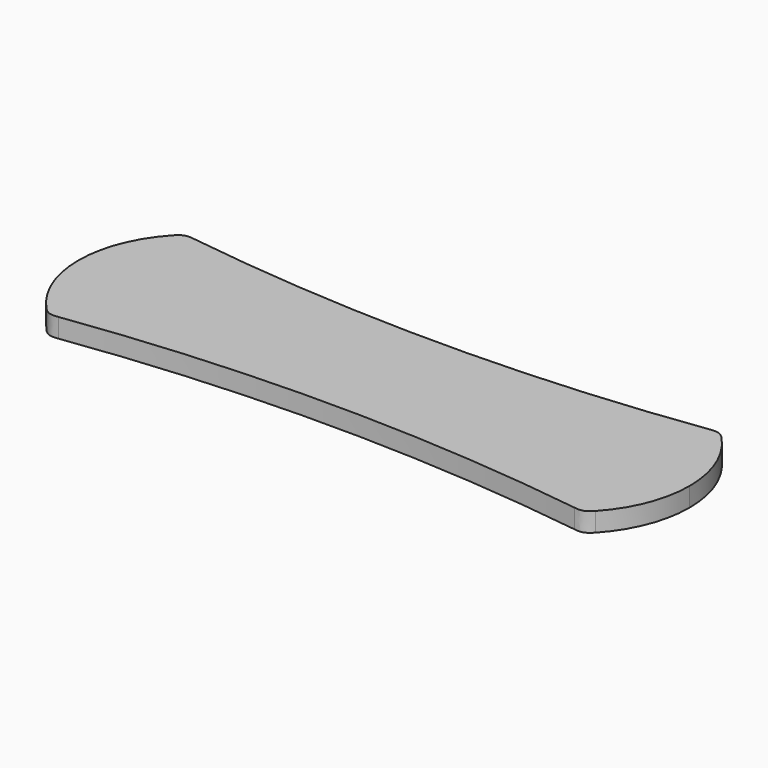
from build123d import *

# Parameters (mm, degrees)
F1_DEPTH    = 25.4
F2_T1_DEPTH = 93.9988541888


# Not quite as in the source:
# - a fillet or chamfer that OpenCascade refuses, or shapes differently, is made with other operations: its cross-section is extruded or revolved along the edge and cut away or added


with BuildPart() as f1:
    # F0 (on Top) → F1 (new body)
    with BuildSketch(Plane.XY):
        with BuildLine():
            ThreePointArc((50.8, 558.8), (13.2719441568, 507.0402470414), (0, 444.5))
            ThreePointArc((0, 444.5), (13.2719441568, 381.9597529586), (50.8, 330.2))
            Line((50.8, 330.2), (50.8, 558.8))
        make_face()
        with BuildLine():
            ThreePointArc((277.2968022896, 536.7332159534), (163.7973759268, 545.1900472484), (50.8, 558.8))
            Line((50.8, 558.8), (50.8, 330.2))
            ThreePointArc((50.8, 330.2), (163.7973759268, 343.8099527516), (277.2968022896, 352.2667840466))
            ThreePointArc((277.2968022896, 352.2667840466), (300.1043048901, 395.8992851393), (307.975, 444.5))
            ThreePointArc((307.975, 444.5), (300.1043048901, 493.1007148607), (277.2968022896, 536.7332159534))
        make_face()
        with BuildLine():
            Line((762, 330.2), (762, 558.8))
            ThreePointArc((762, 558.8), (649.0026240732, 545.1900472484), (535.5031977104, 536.7332159534))
            ThreePointArc((535.5031977104, 536.7332159534), (504.825, 444.5), (535.5031977104, 352.2667840466))
            ThreePointArc((535.5031977104, 352.2667840466), (649.0026240732, 343.8099527516), (762, 330.2))
        make_face()
        with BuildLine():
            ThreePointArc((812.8, 444.5), (799.5280558432, 507.0402470414), (762, 558.8))
            Line((762, 558.8), (762, 330.2))
            ThreePointArc((762, 330.2), (799.5280558432, 381.9597529586), (812.8, 444.5))
        make_face()
        with BuildLine():
            ThreePointArc((535.5031977104, 536.7332159534), (406.4, 533.4), (277.2968022896, 536.7332159534))
            ThreePointArc((277.2968022896, 536.7332159534), (300.1043048901, 493.1007148607), (307.975, 444.5))
            ThreePointArc((307.975, 444.5), (300.1043048901, 395.8992851393), (277.2968022896, 352.2667840466))
            ThreePointArc((277.2968022896, 352.2667840466), (406.4, 355.6), (535.5031977104, 352.2667840466))
            ThreePointArc((535.5031977104, 352.2667840466), (504.825, 444.5), (535.5031977104, 536.7332159534))
        make_face()
    extrude(amount=F1_DEPTH)

    # F2: fillet of radius 25.4 on 4 edges, made by hand

    # F2_s2 → F2_t1 (cut)
    with BuildSketch(Plane.XY.offset(-34.2994270944)):
        with BuildLine():
            add(Edge.make_bspline(
                [(771.7640751065, 549.1617974106), (762.7642490879, 558.8744580913), (749.6481348223, 557.0578149138)],
                knots=[0, 0, 0, 1, 1, 1], degree=2, weights=[1, 1.5, 1]))
            ThreePointArc((749.6481348223, 557.0578149138), (755.8251531993, 557.9212093603), (762, 558.8))
            ThreePointArc((762, 558.8), (766.9894323112, 554.0896960119), (771.7640751065, 549.1617974106))
        make_face()
        with BuildLine():
            add(Edge.make_bspline(
                [(41.0359248935, 549.1617974105), (50.0357509121, 558.8744580913), (63.1518651777, 557.0578149137)],
                knots=[0, 0, 0, 1, 1, 1], degree=2, weights=[1, 1.5, 1]))
            ThreePointArc((63.1518651777, 557.0578149137), (56.9748468007, 557.9212093602), (50.8, 558.8))
            ThreePointArc((50.8, 558.8), (45.8105676888, 554.0896960119), (41.0359248935, 549.1617974105))
        make_face()
        with BuildLine():
            add(Edge.make_bspline(
                [(41.0359248935, 339.8382025894), (50.0357509121, 330.1255419087), (63.1518651777, 331.9421850862)],
                knots=[0, 0, 0, 1, 1, 1], degree=2, weights=[1, 1.5, 1]))
            ThreePointArc((63.1518651777, 331.9421850862), (56.9748468007, 331.0787906397), (50.8, 330.2))
            ThreePointArc((50.8, 330.2), (45.8105676888, 334.9103039881), (41.0359248935, 339.8382025894))
        make_face()
        with BuildLine():
            add(Edge.make_bspline(
                [(749.6481348223, 331.9421850862), (762.7642490879, 330.1255419087), (771.7640751065, 339.8382025894)],
                knots=[0, 0, 0, 1, 1, 1], degree=2, weights=[1, 1.5, 1]))
            ThreePointArc((771.7640751065, 339.8382025894), (766.9894323112, 334.9103039881), (762, 330.2))
            ThreePointArc((762, 330.2), (755.8251531993, 331.0787906397), (749.6481348223, 331.9421850862))
        make_face()
    extrude(amount=F2_T1_DEPTH, mode=Mode.SUBTRACT)


solid = f1.part
